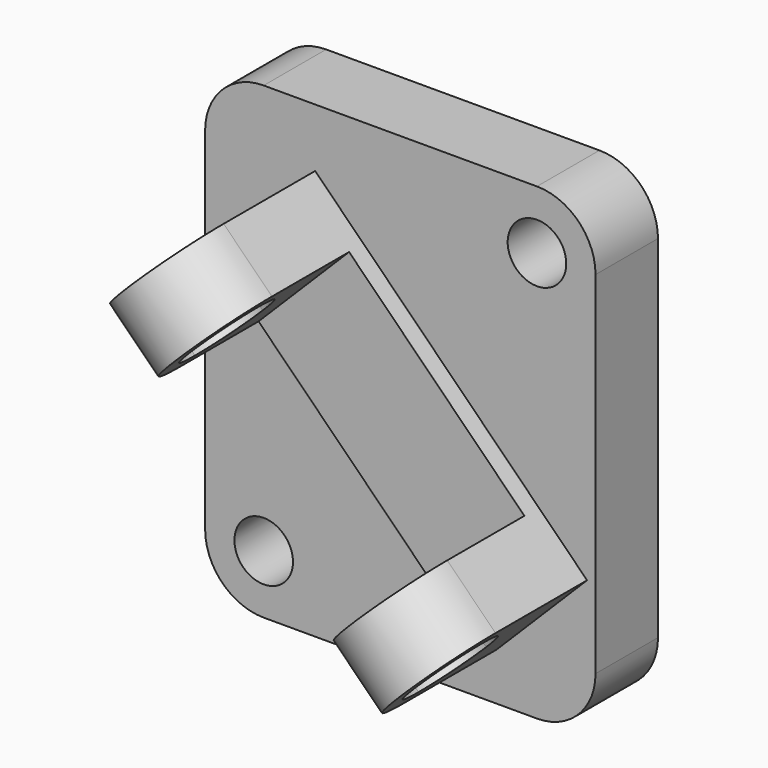
from build123d import *

# Parameters (mm, degrees)
F0_R     = 19.05
F1_DEPTH = 25.4
F2_DEPTH = 99.822
F4_DEPTH = 250.19
F5_DEPTH = 250.19
F6_W     = 161.29
F6_H     = 62.738
F6_H_2   = 49.2019202976
F7_DEPTH = 171.704


# Not quite as in the source:
# - a feature names something its author has since deleted; it is built from what else it names


with BuildPart() as f1:
    # F0 (on Front) → F1 (new body, symmetric)
    with BuildSketch(Plane.XZ):
        with BuildLine():
            ThreePointArc((0, 38.1), (11.1592316368, 11.1592316368), (38.1, 0))
            Line((38.1, 0), (215.9, 0))
            ThreePointArc((215.9, 0), (242.8407683632, 11.1592316368), (254, 38.1))
            Line((254, 38.1), (254, 266.7))
            ThreePointArc((254, 266.7), (242.8407683632, 293.6407683632), (215.9, 304.8))
            Line((215.9, 304.8), (38.1, 304.8))
            ThreePointArc((38.1, 304.8), (11.1592316368, 293.6407683632), (0, 266.7))
            Line((0, 266.7), (0, 38.1))
        make_face()
        with BuildLine():
            ThreePointArc((57.0266099035, 35.9352973504), (37.3773915988, 19.0637099965), (19.0637495923, 37.376349246))
            ThreePointArc((19.0637495923, 37.376349246), (37.7381093173, 57.1465622918), (57.15, 38.1))
            ThreePointArc((57.15, 38.1), (57.1191274598, 37.0158917631), (57.0266099035, 35.9352973504))
        make_face(mode=Mode.SUBTRACT)
        Polygon((248.4933634432, 89.814005202), (189.582883289, 30.9035250478), (12.671837704, 207.8145706329), (71.5823178582, 266.7250507871), align=None, mode=Mode.SUBTRACT)
        with Locations((215.9, 266.7)):
            Circle(F0_R, mode=Mode.SUBTRACT)
        Polygon((12.671837704, 207.8145706329), (189.582883289, 30.9035250478), (248.4933634432, 89.814005202), (71.5823178582, 266.7250507871), align=None)
    extrude(amount=F1_DEPTH, both=True)

    # F0 (on Front) → F2 (join)
    with BuildSketch(Plane.XZ):
        Polygon((12.671837704, 207.8145706329), (189.582883289, 30.9035250478), (248.4933634432, 89.814005202), (71.5823178582, 266.7250507871), align=None)
    extrude(amount=F2_DEPTH)

    # F3 (on face) → F4 (join)
    with BuildSketch(Plane(origin=(79.3396791206, 0, -79.3396791206), x_dir=(0, 1, 0), z_dir=(0.7071067812, 0, -0.7071067812))):
        with BuildLine():
            ThreePointArc((-99.822, 168.3534344944), (-129.032, 197.5634344944), (-99.822, 226.7734344944))
            Line((-99.822, 226.7734344944), (-99.822, 239.2194344944))
            ThreePointArc((-99.822, 239.2194344944), (-141.478, 197.5634344944), (-99.822, 155.9074344944))
            Line((-99.822, 155.9074344944), (-99.822, 168.3534344944))
        make_face()
    extrude(amount=-F4_DEPTH)

    # F3 (on face) → F5 (cut)
    with BuildSketch(Plane(origin=(79.3396791206, 0, -79.3396791206), x_dir=(0, 1, 0), z_dir=(0.7071067812, 0, -0.7071067812))):
        with BuildLine():
            ThreePointArc((-99.822, 168.3534344944), (-79.1674109215, 176.908845416), (-70.612, 197.5634344944))
            ThreePointArc((-70.612, 197.5634344944), (-79.1674109215, 218.2180235729), (-99.822, 226.7734344944))
            Line((-99.822, 226.7734344944), (-99.822, 168.3534344944))
        make_face()
    extrude(amount=-F5_DEPTH, mode=Mode.SUBTRACT)

    # F6 (on face) → F7 (cut)
    with BuildSketch(Plane(origin=(110.2432041684, 0, 110.2432041684), x_dir=(0.7071067812, 0, -0.7071067812), z_dir=(-0.7071067812, 0, -0.7071067812))):
        with Locations((-12.8917497533, 68.453)):
            Rectangle(F6_W, F6_H)
        with Locations((-12.8917497533, 124.4229601488)):
            Rectangle(F6_W, F6_H_2)
    extrude(amount=-F7_DEPTH, mode=Mode.SUBTRACT)


solid = f1.part
